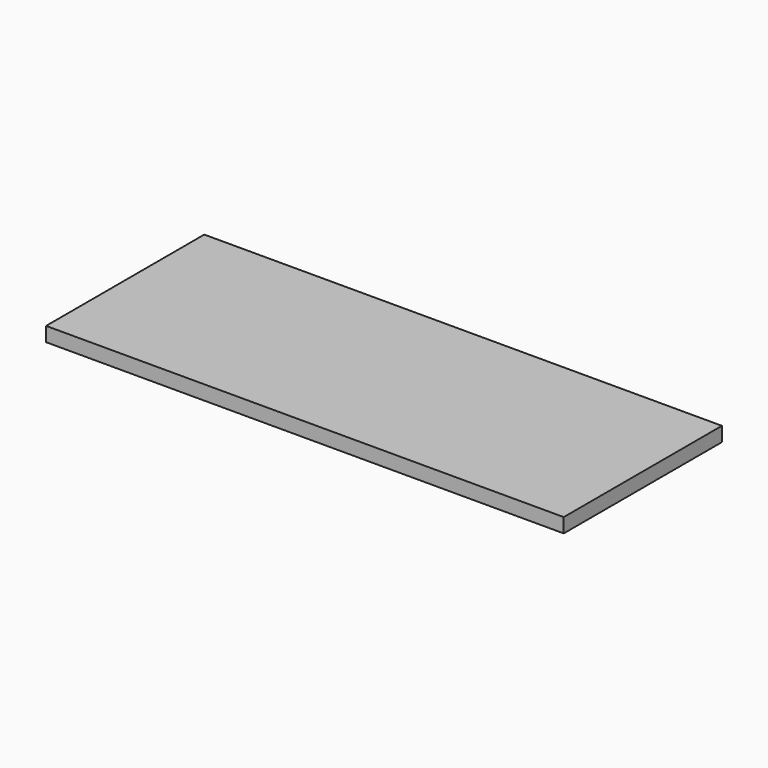
from build123d import *

# Parameters (mm, degrees)
F0_W     = 914.4
F0_H     = 349.25
F1_DEPTH = 12.7
F2_W     = 863.6
F2_H     = 12.7
F3_DEPTH = 12.7
F4_W     = 9.525
F4_H     = 304.8
F5_DEPTH = 12.7


# Not quite as in the source:
# - a feature names something its author has since deleted; it is built from what else it names


with BuildPart() as f1:
    # F0 (on Top) → F1 (new body, symmetric)
    with BuildSketch(Plane.XY):
        Rectangle(F0_W, F0_H)
    extrude(amount=F1_DEPTH, both=True)

    # F2 (on face) → F3 (cut)
    with BuildSketch(Plane(origin=(0, 0, -12.7), x_dir=(1, 0, 0), z_dir=(0, 0, -1))):
        with Locations((0, 155.575)):
            Rectangle(F2_W, F2_H)
    extrude(amount=-F3_DEPTH, mode=Mode.SUBTRACT)

    # F4 (on face) → F5 (cut)
    with BuildSketch(Plane(origin=(0, 0, -12.7), x_dir=(1, 0, 0), z_dir=(0, 0, -1))):
        with Locations((-436.5625, -9.525)):
            Rectangle(F4_W, F4_H)
        with Locations((436.5625, -9.525)):
            Rectangle(F4_W, F4_H)
    extrude(amount=-F5_DEPTH, mode=Mode.SUBTRACT)


solid = f1.part
